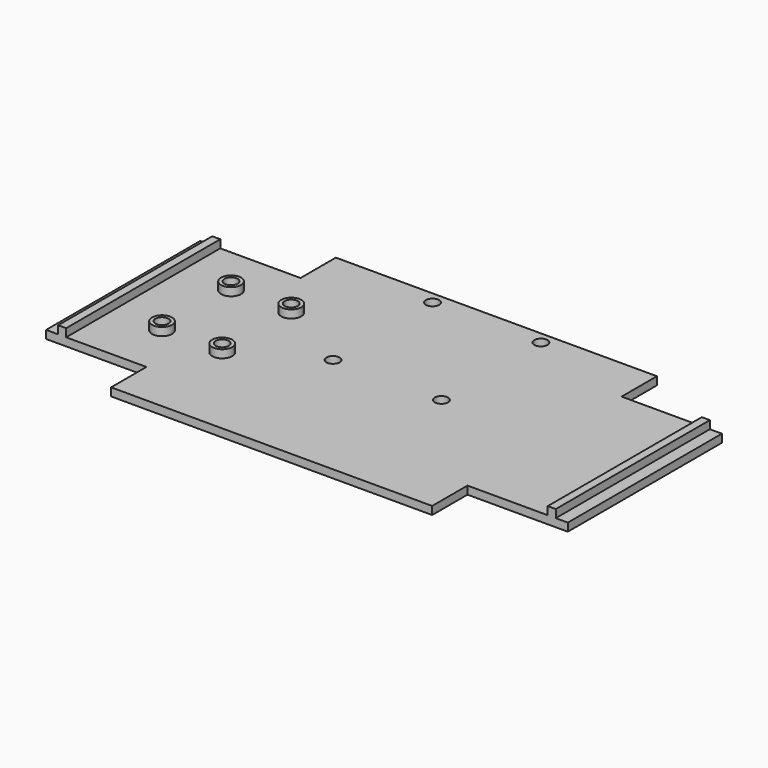
from build123d import *

# Parameters (mm, degrees)
F0_R     = 2.5
F0_W     = 20
F0_H     = 48
F0_W_2   = 3
F0_W_3   = 2
F1_DEPTH = 2
F2_DEPTH = 2
F3_D     = 3.3
F3_DEPTH = 2.001
F4_D     = 3.3


# Not quite as in the source:
# - a feature names something its author has since deleted; it is built from what else it names


with BuildPart() as f1:
    # F0 (on Top) → F1 (new body)
    with BuildSketch(Plane.XY):
        Polygon((-17.7864517868, 26.073888598), (-50.0104304813, 26.073888598), (-50.0104304813, -21.926111402), (-17.7864517868, -21.926111402), (19.2135482132, -21.926111402), (29.9895695187, -21.926111402), (29.9895695187, 26.073888598), (19.2135482132, 26.073888598), align=None)
        with Locations((-42.2986224294, -7.9553306252)):
            Circle(F0_R, mode=Mode.SUBTRACT)
        with Locations((-42.2986224294, 13.5446693748)):
            Circle(F0_R, mode=Mode.SUBTRACT)
        Polygon((-50.0104304813, -21.926111402), (-50.0104304813, 26.073888598), (-54.2864517868, 26.073888598), (-70.0104304813, 26.073888598), (-70.0104304813, -21.926111402), (-54.2864517868, -21.926111402), align=None)
        with Locations((-57.2986224294, -7.9553306252)):
            Circle(F0_R, mode=Mode.SUBTRACT)
        with Locations((-57.2986224294, 13.5446693748)):
            Circle(F0_R, mode=Mode.SUBTRACT)
        with Locations((39.9895695187, 2.073888598)):
            Rectangle(F0_W, F0_H)
        Polygon((29.9895695187, 37.073888598), (-50.0104304813, 37.073888598), (-50.0104304813, 26.073888598), (-17.7864517868, 26.073888598), (19.2135482132, 26.073888598), (29.9895695187, 26.073888598), align=None)
        Polygon((-17.7864517868, -21.926111402), (-50.0104304813, -21.926111402), (-50.0104304813, -32.926111402), (29.9895695187, -32.926111402), (29.9895695187, -21.926111402), (19.2135482132, -21.926111402), align=None)
        with Locations((-73.5104304813, 2.073888598)):
            Rectangle(F0_W_2, F0_H)
        with Locations((53.4895695187, 2.073888598)):
            Rectangle(F0_W_2, F0_H)
        with Locations((-71.0104304813, 2.073888598)):
            Rectangle(F0_W_3, F0_H)
        with Locations((50.9895695187, 2.073888598)):
            Rectangle(F0_W_3, F0_H)
        with Locations((-42.2986224294, 13.5446693748)):
            Circle(F0_R)
        with Locations((-42.2986224294, -7.9553306252)):
            Circle(F0_R)
        with Locations((-57.2986224294, -7.9553306252)):
            Circle(F0_R)
        with Locations((-57.2986224294, 13.5446693748)):
            Circle(F0_R)
    extrude(amount=-F1_DEPTH)

    # F0 (on Top) → F2 (join)
    with BuildSketch(Plane.XY):
        with Locations((-71.0104304813, 2.073888598)):
            Rectangle(F0_W_3, F0_H)
        with Locations((50.9895695187, 2.073888598)):
            Rectangle(F0_W_3, F0_H)
        with Locations((-57.2986224294, 13.5446693748)):
            Circle(F0_R)
        with Locations((-42.2986224294, 13.5446693748)):
            Circle(F0_R)
        with Locations((-42.2986224294, -7.9553306252)):
            Circle(F0_R)
        with Locations((-57.2986224294, -7.9553306252)):
            Circle(F0_R)
    extrude(amount=F2_DEPTH)

    # F3 (through all, one way)
    with BuildSketch(Plane.XY):
        with Locations((-23.5104304813, 3.073888598), (3.4895695187, 3.073888598), (3.4895695187, 34.073888598), (-23.5104304813, 34.073888598), (-57.2986224294, 13.5446693748), (-42.2986224294, 13.5446693748), (-42.2986224294, -7.9553306252), (-57.2986224294, -7.9553306252)):
            Circle(F3_D / 2)
    extrude(amount=-F3_DEPTH, mode=Mode.SUBTRACT)

    # F4 (through all)
    with Locations(Plane(origin=(0, 0, 0), x_dir=(1, 0, 0), z_dir=(0, 0, -1))):
        with Locations((-57.2986224294, -13.5446693748), (-57.2986224294, 7.9553306252), (-42.2986224294, -13.5446693748), (-42.2986224294, 7.9553306252)):
            Hole(F4_D / 2)


solid = f1.part
